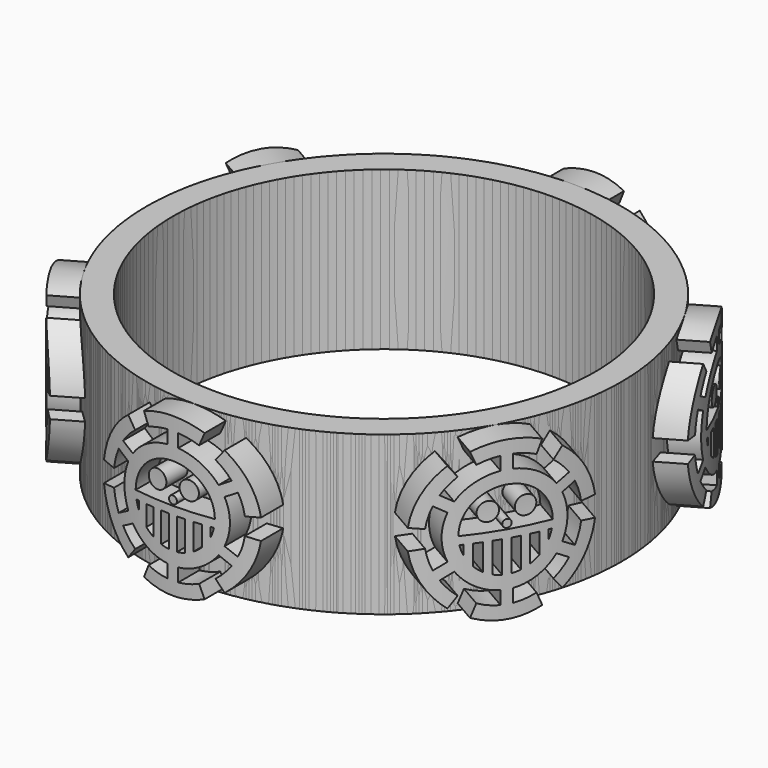
from build123d import *
from build123d import SkipClean  # not in build123d's __all__

# Parameters (mm, degrees)
F0_R      = 3.81
F1_DEPTH  = 13.97
F2_R      = 0.4445
F2_R_2    = 0.1905
F3_DEPTH  = 50.8
F4_R      = 11.43
F4_R_2    = 10.16
F5_DEPTH  = 7.62
F6_R      = 16.7893257343
F6_R_2    = 12.7
F7_DEPTH  = 7.6210001
F8_R      = 10.16
F9_DEPTH  = 7.6210001
F11_COUNT = 6


with BuildPart() as f1:
    # F0 (on Front) → F1 (new body)
    with BuildSketch(Plane.XZ):
        with Locations((0, 3.81)):
            Circle(F0_R)
    extrude(amount=F1_DEPTH)

    # F2 (on face) → F3 (cut)
    with BuildSketch(Plane.XZ.offset(13.97)):
        with BuildLine():
            Line((-2.3193810445, 6.8326762265), (-1.9328175371, 6.3288968554))
            ThreePointArc((-1.9328175371, 6.3288968554), (-2.3013737871, 5.997305121), (-2.6138177156, 5.6123822984))
            Line((-2.6138177156, 5.6123822984), (-2.0616783683, 5.2936044977))
            ThreePointArc((-2.0616783683, 5.2936044977), (-1.27, 6.0097045256), (-0.254, 6.3372680903))
            Line((-0.254, 6.3372680903), (-0.254, 6.9748236918))
            ThreePointArc((-0.254, 6.9748236918), (-0.743574907, 6.8967007237), (-1.2150198978, 6.7433175157))
            Line((-1.2150198978, 6.7433175157), (-1.4580238773, 7.3299810189))
            ThreePointArc((-1.4580238773, 7.3299810189), (-1.905, 7.1095567884), (-2.3193810445, 6.8326762265))
        make_face()
        with BuildLine():
            ThreePointArc((2.3193810445, 6.8326762265), (1.905, 7.1095567884), (1.4580238773, 7.3299810189))
            Line((1.4580238773, 7.3299810189), (1.2150198978, 6.7433175157))
            ThreePointArc((1.2150198978, 6.7433175157), (0.743574907, 6.8967007237), (0.254, 6.9748236918))
            Line((0.254, 6.9748236918), (0.254, 6.3372680903))
            ThreePointArc((0.254, 6.3372680903), (1.27, 6.0097045256), (2.0616783683, 5.2936044977))
            Line((2.0616783683, 5.2936044977), (2.6138177156, 5.6123822984))
            ThreePointArc((2.6138177156, 5.6123822984), (2.3013737871, 5.997305121), (1.9328175371, 6.3288968554))
            Line((1.9328175371, 6.3288968554), (2.3193810445, 6.8326762265))
        make_face()
        with BuildLine():
            Line((-3.1478374349, 4.2244206603), (-3.7774049218, 4.3073047924))
            ThreePointArc((-3.7774049218, 4.3073047924), (-3.81, 3.81), (-3.7774049218, 3.3126952076))
            Line((-3.7774049218, 3.3126952076), (-3.1478374349, 3.3955793397))
            ThreePointArc((-3.1478374349, 3.3955793397), (-3.0449486941, 2.9106043973), (-2.8678177156, 2.4475586067))
            Line((-2.8678177156, 2.4475586067), (-2.3156783683, 2.7663364074))
            ThreePointArc((-2.3156783683, 2.7663364074), (-2.54, 3.81), (-2.3156783683, 4.8536635926))
            Line((-2.3156783683, 4.8536635926), (-2.8678177156, 5.1724413933))
            ThreePointArc((-2.8678177156, 5.1724413933), (-3.0449486941, 4.7093956027), (-3.1478374349, 4.2244206603))
        make_face()
        with BuildLine():
            Line((-1.9328175371, 1.2911031446), (-2.3193810445, 0.7873237735))
            ThreePointArc((-2.3193810445, 0.7873237735), (-1.905, 0.5104432116), (-1.4580238773, 0.2900189811))
            Line((-1.4580238773, 0.2900189811), (-1.2150198978, 0.8766824843))
            ThreePointArc((-1.2150198978, 0.8766824843), (-0.743574907, 0.7232992763), (-0.254, 0.6451763082))
            Line((-0.254, 0.6451763082), (-0.254, 1.2827319097))
            ThreePointArc((-0.254, 1.2827319097), (-1.27, 1.6102954744), (-2.0616783683, 2.3263955023))
            Line((-2.0616783683, 2.3263955023), (-2.6138177156, 2.0076177016))
            ThreePointArc((-2.6138177156, 2.0076177016), (-2.3013737871, 1.622694879), (-1.9328175371, 1.2911031446))
        make_face()
        with BuildLine():
            Line((1.2150198978, 0.8766824843), (1.4580238773, 0.2900189811))
            ThreePointArc((1.4580238773, 0.2900189811), (1.905, 0.5104432116), (2.3193810445, 0.7873237735))
            Line((2.3193810445, 0.7873237735), (1.9328175371, 1.2911031446))
            ThreePointArc((1.9328175371, 1.2911031446), (2.3013737871, 1.622694879), (2.6138177156, 2.0076177016))
            Line((2.6138177156, 2.0076177016), (2.0616783683, 2.3263955023))
            ThreePointArc((2.0616783683, 2.3263955023), (1.27, 1.6102954744), (0.254, 1.2827319097))
            Line((0.254, 1.2827319097), (0.254, 0.6451763082))
            ThreePointArc((0.254, 0.6451763082), (0.743574907, 0.7232992763), (1.2150198978, 0.8766824843))
        make_face()
        with BuildLine():
            ThreePointArc((3.81, 3.81), (3.8018424975, 4.0591859224), (3.7774049218, 4.3073047924))
            Line((3.7774049218, 4.3073047924), (3.1478374349, 4.2244206603))
            ThreePointArc((3.1478374349, 4.2244206603), (3.0449486941, 4.7093956027), (2.8678177156, 5.1724413933))
            Line((2.8678177156, 5.1724413933), (2.3156783683, 4.8536635926))
            ThreePointArc((2.3156783683, 4.8536635926), (2.54, 3.81), (2.3156783683, 2.7663364074))
            Line((2.3156783683, 2.7663364074), (2.8678177156, 2.4475586067))
            ThreePointArc((2.8678177156, 2.4475586067), (3.0449486941, 2.9106043973), (3.1478374349, 3.3955793397))
            Line((3.1478374349, 3.3955793397), (3.7774049218, 3.3126952076))
            ThreePointArc((3.7774049218, 3.3126952076), (3.8018424975, 3.5608140776), (3.81, 3.81))
        make_face()
        with BuildLine():
            Line((-1.7145, 3.429), (-1.866511184, 3.429))
            ThreePointArc((-1.866511184, 3.429), (-1.8045480543, 3.1995646472), (-1.7145, 2.9796297513))
            Line((-1.7145, 2.9796297513), (-1.7145, 3.429))
        make_face()
        with BuildLine():
            Line((-0.9525, 2.1602216058), (-0.9525, 3.429))
            Line((-0.9525, 3.429), (-1.3335, 3.429))
            Line((-1.3335, 3.429), (-1.3335, 2.4495578844))
            ThreePointArc((-1.3335, 2.4495578844), (-1.1521188613, 2.2928819659), (-0.9525, 2.1602216058))
        make_face()
        with BuildLine():
            Line((-0.1905, 1.9145489323), (-0.1905, 3.429))
            Line((-0.1905, 3.429), (-0.5715, 3.429))
            Line((-0.5715, 3.429), (-0.5715, 1.9927458213))
            ThreePointArc((-0.5715, 1.9927458213), (-0.3830008986, 1.9438983651), (-0.1905, 1.9145489323))
        make_face()
        with BuildLine():
            Line((0.5715, 3.429), (0.1905, 3.429))
            Line((0.1905, 3.429), (0.1905, 1.9145489323))
            ThreePointArc((0.1905, 1.9145489323), (0.3830008986, 1.9438983651), (0.5715, 1.9927458213))
            Line((0.5715, 1.9927458213), (0.5715, 3.429))
        make_face()
        with BuildLine():
            Line((1.3335, 3.429), (0.9525, 3.429))
            Line((0.9525, 3.429), (0.9525, 2.1602216058))
            ThreePointArc((0.9525, 2.1602216058), (1.1521188613, 2.2928819659), (1.3335, 2.4495578844))
            Line((1.3335, 2.4495578844), (1.3335, 3.429))
        make_face()
        with BuildLine():
            ThreePointArc((1.905, 3.81), (0, 5.715), (-1.905, 3.81))
            Line((-1.905, 3.81), (1.905, 3.81))
        make_face()
        with Locations((-0.762, 4.699)):
            Circle(F2_R, mode=Mode.SUBTRACT)
        with Locations((0, 4.064)):
            Circle(F2_R_2, mode=Mode.SUBTRACT)
        with Locations((0.762, 4.699)):
            Circle(F2_R, mode=Mode.SUBTRACT)
        with BuildLine():
            Line((1.866511184, 3.429), (1.7145, 3.429))
            Line((1.7145, 3.429), (1.7145, 2.9796297513))
            ThreePointArc((1.7145, 2.9796297513), (1.8045480543, 3.1995646472), (1.866511184, 3.429))
        make_face()
    extrude(amount=-F3_DEPTH, mode=Mode.SUBTRACT)

    # F4 (on Top) → F5 (join)
    with BuildSketch(Plane.XY):
        Circle(F4_R)
        Circle(F4_R_2, mode=Mode.SUBTRACT)
    with SkipClean():  # cleaning this boolean's faces spoils the solid; the shape is the same uncleaned
        extrude(amount=F5_DEPTH)

    # F6 (on face) → F7 (cut, through all)
    with BuildSketch(Plane.XY.offset(7.62)):
        Circle(F6_R)
        Circle(F6_R_2, mode=Mode.SUBTRACT)
    with SkipClean():  # cleaning this boolean's faces spoils the solid; the shape is the same uncleaned
        extrude(amount=-F7_DEPTH, mode=Mode.SUBTRACT)

    # F8 (on face) → F9 (cut, through all)
    with BuildSketch(Plane.XY.offset(7.62)):
        Circle(F8_R)
    with SkipClean():  # cleaning this boolean's faces spoils the solid; the shape is the same uncleaned
        extrude(amount=-F9_DEPTH, mode=Mode.SUBTRACT)


with BuildPart() as f11_1:
    # F11: instance of F1
    add(f1.part.rotate(Axis((0, 0, 16.905374825), (0, 0, 1)), 1 * 360 / F11_COUNT), clean=False)


with BuildPart() as f11_2:
    # F11: instance of F1
    add(f1.part.rotate(Axis((0, 0, 16.905374825), (0, 0, 1)), 2 * 360 / F11_COUNT), clean=False)


with BuildPart() as f11_3:
    # F11: instance of F1
    add(f1.part.rotate(Axis((0, 0, 16.905374825), (0, 0, 1)), 3 * 360 / F11_COUNT), clean=False)


with BuildPart() as f11_4:
    # F11: instance of F1
    add(f1.part.rotate(Axis((0, 0, 16.905374825), (0, 0, 1)), 4 * 360 / F11_COUNT), clean=False)


with BuildPart() as f11_5:
    # F11: instance of F1
    add(f1.part.rotate(Axis((0, 0, 16.905374825), (0, 0, 1)), 5 * 360 / F11_COUNT), clean=False)


solid = Compound([f1.part, f11_1.part, f11_2.part, f11_3.part, f11_4.part, f11_5.part])
